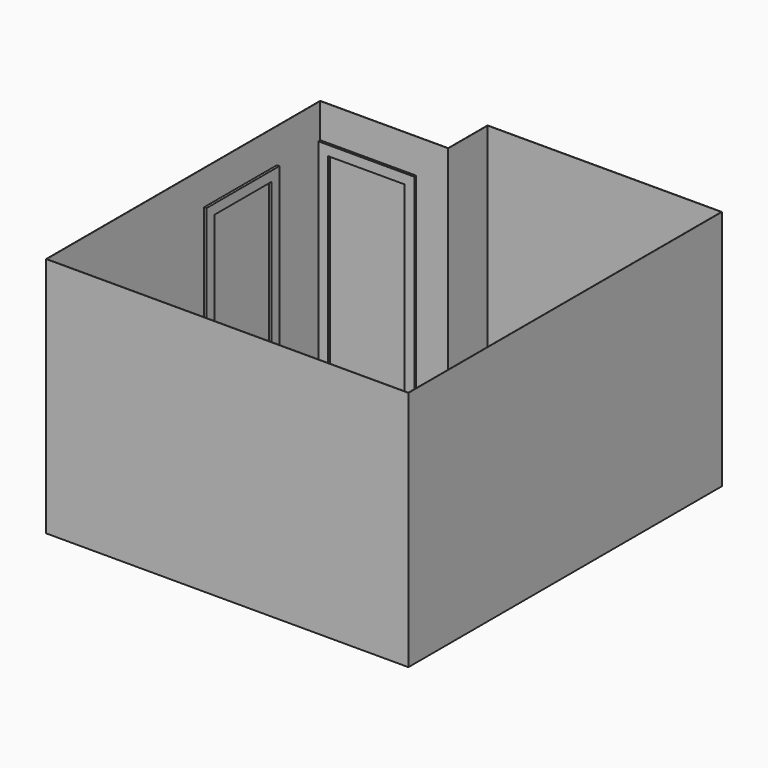
from build123d import *

# Parameters (mm, degrees)
F1_DEPTH = 2489.2
F2_T     = 2.54
F4_DEPTH = 25.4
F6_DEPTH = 25.4
F8_DEPTH = 25.4


with BuildPart() as f1:
    # F0 (on Top) → F1 (new body)
    with BuildSketch(Plane.XY):
        Polygon((0, 3530.6), (0, 0), (3733.8, 0), (3733.8, 4038.6), (1320.8, 4038.6), (1320.8, 3530.6), align=None)
    extrude(amount=F1_DEPTH)

    # F2
    f2_openings = [f1.faces().sort_by_distance(p)[0] for p in [
        (1923.084122, 1937.093758, 2489.2),
    ]]
    offset(amount=F2_T, openings=f2_openings, kind=Kind.INTERSECTION)

    # F3 (on face) → F4 (join)
    with BuildSketch(Plane(origin=(3733.8, 0, 0), x_dir=(0, -1, 0), z_dir=(-1, 0, 0))):
        Polygon((-3987.8, 2133.6), (-3987.8, 0), (-3886.2, 0), (-3886.2, 2032), (-3098.8, 2032), (-3098.8, 0), (-2997.2, 0), (-2997.2, 2133.6), align=None)
    extrude(amount=F4_DEPTH)

    # F5 (on face) → F6 (join)
    with BuildSketch(Plane.XZ.offset(-3530.6)):
        Polygon((0, 2133.6), (0, 0), (101.6, 0), (101.6, 2032), (889, 2032), (889, 0), (990.6, 0), (990.6, 2133.6), align=None)
    extrude(amount=F6_DEPTH)

    # F7 (on face) → F8 (join)
    with BuildSketch(Plane.YZ):
        Polygon((2032, 2133.6), (2032, 0), (2133.6, 0), (2133.6, 2032), (2870.2, 2032), (2870.2, 0), (2971.8, 0), (2971.8, 2133.6), align=None)
    extrude(amount=F8_DEPTH)


solid = f1.part
